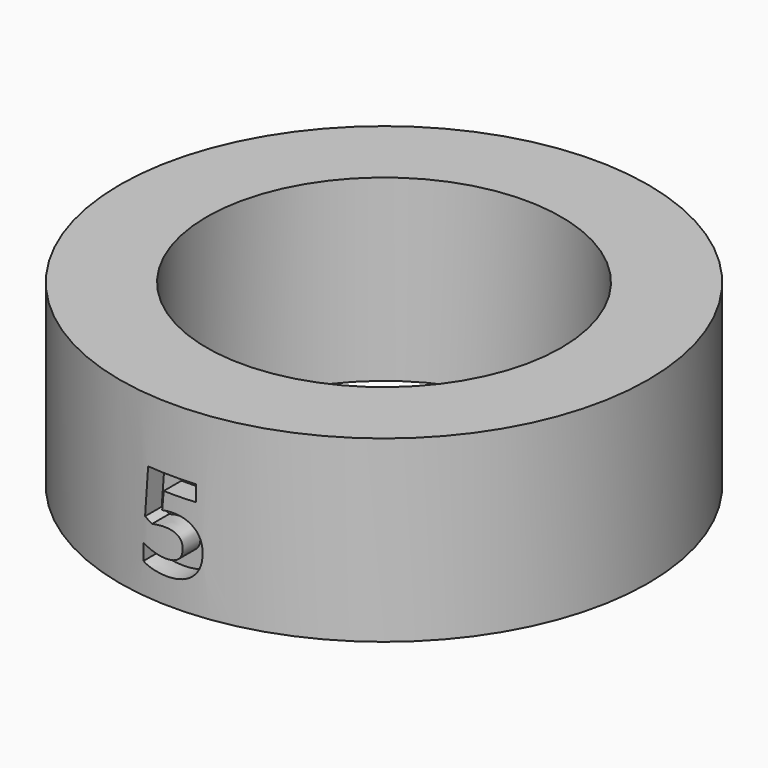
from build123d import *

# Parameters (mm, degrees)
F0_R         = 14.75
F0_R_2       = 9.9
F1_DEPTH     = 10
F3_TEXT_SIZE = 6.9444444444
F4_DEPTH     = 1.5


# Not quite as in the source:
# - Text() gives the source's letters only with a copy of the font that has no kerning and outlines rounded to 1/6400 em; it was checked with that copy


with BuildPart() as f1:
    # F0 (on Top) → F1 (new body)
    with BuildSketch(Plane.XY):
        Circle(F0_R)
        Circle(F0_R_2, mode=Mode.SUBTRACT)
    extrude(amount=F1_DEPTH)

    # F3 (on offset) → F4 (cut)
    with BuildSketch(Plane.XZ.offset(15)):
        with Locations((-2.0513237847, 1.500000013)):
            Text('5', F3_TEXT_SIZE, font='Open Sans', font_style=FontStyle.BOLD, text_align=(TextAlign.LEFT, TextAlign.BOTTOM))
    extrude(amount=-F4_DEPTH, mode=Mode.SUBTRACT)


solid = f1.part
